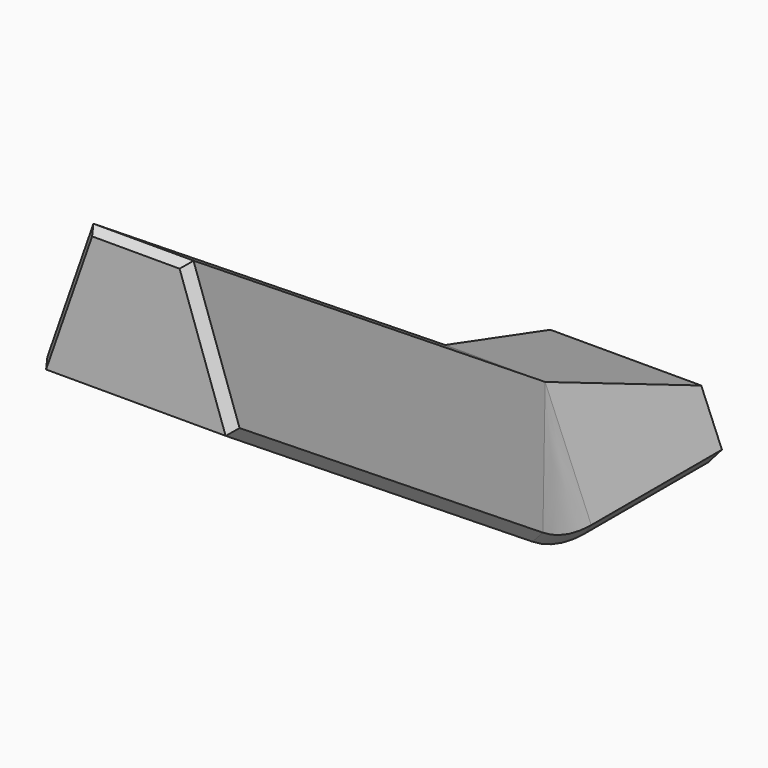
from build123d import *

# Parameters (mm, degrees)
F1_DEPTH  = 8
F3_ANGLE  = 33
F6_DEPTH  = 26.5
F7_W      = 18.4942251071
F7_H      = 9.6429027617
F8_DEPTH  = 25
F9_SIZE   = 0.5
F10_SIZE2 = 2.99999
F10_SIZE  = 7.99999
F11_SIZE  = 0.46
F12_SIZE  = 0.475
F13_SIZE  = 0.56


# Not quite as in the source:
# - a fillet or chamfer is up to 0.001 mm smaller than in the source, because OpenCascade refuses the exact size


with BuildPart() as f1:
    # F0 (on Front) → F1 (new body)
    with BuildSketch(Plane.XZ):
        Polygon((-2.45, 5.9), (-4.9, 0), (4.9, 0), (2.45, 5.9), align=None)
    extrude(amount=F1_DEPTH)

    # F2 (on face) → F3 (revolve)
    with BuildSketch(Plane.XZ.offset(8)):
        Polygon((4.9, 0), (2.45, 5.9), (-2.45, 5.9), (-4.9, 0), align=None)
    revolve(axis=Axis((0, -8, 5.9), (-1, 0, 0)), revolution_arc=F3_ANGLE)

    # F4 (on face) → F6 (join)
    with BuildSketch(Plane(origin=(0, -8.3219056723, 5.4043087335), x_dir=(1, 0, 0), z_dir=(0, -0.8386705679, 0.544639035))):
        Polygon((-4.9, -5.3089559292), (4.9, -5.3089559292), (2.45, 0.5910440708), (-2.45, 0.5910440708), align=None)
    extrude(amount=F6_DEPTH)

    # F7 (on Top) → F8 (cut)
    with BuildSketch(Plane.XY):
        with Locations((0.8348836564, -34.8214513808)):
            Rectangle(F7_W, F7_H)
    extrude(amount=F8_DEPTH, mode=Mode.SUBTRACT)

    # F9
    f9_edges = [f1.edges().sort_by_distance(p)[0] for p in [
        (4.9, -4, 0),
        (-4.9, -4, 0),
    ]]
    chamfer(f9_edges, length=F9_SIZE)

    # F10 (size 8 and 3 in the source; OpenCascade refuses exactly that, so slightly less here)
    f10_edges = [f1.edges().sort_by_distance(p)[0] for p in [
        (0, 0, 5.9),
    ]]
    f10_side = f1.faces().sort_by_distance((0, -4, 5.9))[0]
    chamfer(f10_edges, length=F10_SIZE, length2=F10_SIZE2, reference=f10_side)

    # F11
    f11_edges = [f1.edges().sort_by_distance(p)[0] for p in [
        (0, 0, 0),
    ]]
    chamfer(f11_edges, length=F11_SIZE)

    # F12
    f12_edges = [f1.edges().sort_by_distance(p)[0] for p in [
        (-3.579124, -30, 16.944794),
        (3.579124, -30, 16.944794),
    ]]
    chamfer(f12_edges, length=F12_SIZE)

    # F13
    f13_edges = [f1.edges().sort_by_distance(p)[0] for p in [
        (0, -30, 20.186967),
    ]]
    chamfer(f13_edges, length=F13_SIZE)


solid = f1.part
